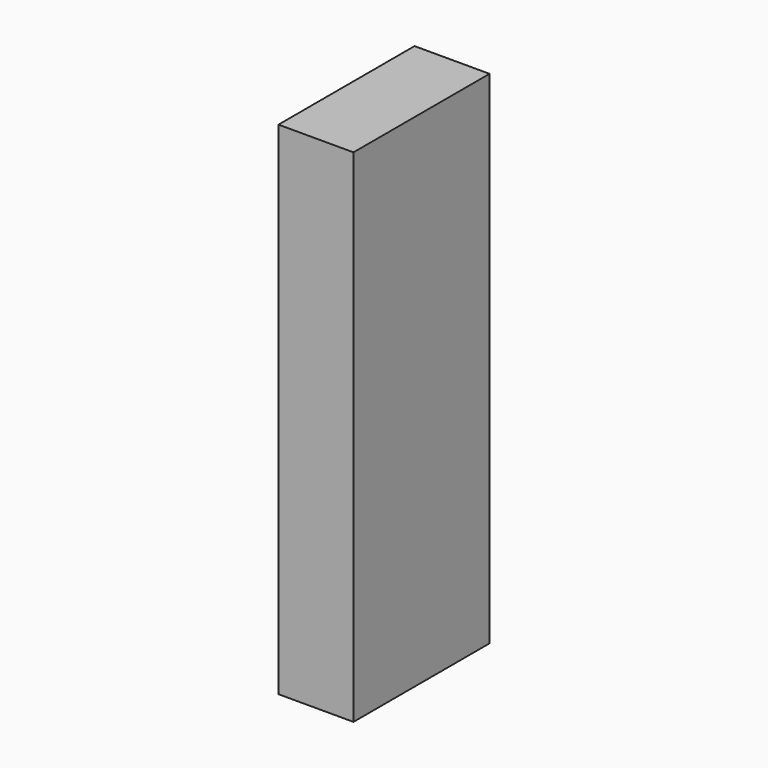
from build123d import *

# Parameters (mm, degrees)
F1_DEPTH = 64617.6


# Not quite as in the source:
# - the program builds the solid bodies; features that only make, move or delete a surface that nothing else refers to are left out


with BuildPart() as f1:
    # F0 (on Front) → F1 (new body, symmetric)
    with BuildSketch(Plane.XZ):
        Polygon((-56997.6, 0), (0, 0), (0, 381000), (-28498.8, 381000), (-56997.6, 381000), align=None)
    extrude(amount=F1_DEPTH, both=True)


solid = f1.part
